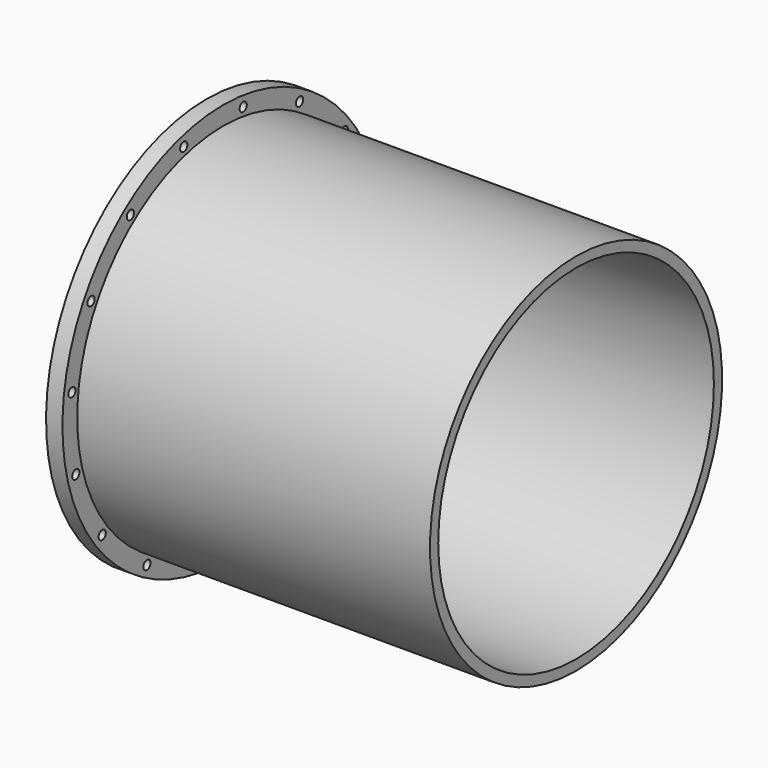
from build123d import *

# Parameters (mm, degrees)
F0_W            = 790
F0_H            = 6
F2_W            = 790
F2_H            = 8
F5_D            = 22
F5_COPIES_COUNT = 16


# Not quite as in the source:
# - a pattern or mirror of a feature is missing from the dataset's text; its kind, count and spacing are read off the source's solid


with BuildPart() as f1:
    # F0 (on Front) → F1 (revolve)
    with BuildSketch(Plane.XZ):
        Polygon((-450, 490), (-450, 420), (450, 420), (450, 445), (-410, 445), (-410, 490), align=None)
        with Locations((-15, 435)):
            Rectangle(F0_W, F0_H, mode=Mode.SUBTRACT)
    revolve(axis=Axis((-71.5964585543, 0, 0), (1, 0, 0)))

    # F2 (on Front) → F3 (revolve, cut)
    with BuildSketch(Plane.XZ):
        with Locations((-15, 434)):
            Rectangle(F2_W, F2_H)
    revolve(axis=Axis((-160.7926189899, 0, 0), (1, 0, 0)), mode=Mode.SUBTRACT)

    # F5 (through all)
    with Locations(Plane(origin=(-450, 0, 0), x_dir=(0, -1, 0), z_dir=(-1, 0, 0))):
        with Locations((-232.5, 402.7018127598)):
            f5 = Hole(F5_D / 2)

    # F5_copies: F5 ×16 about axis
    f5_copies_axis = Axis((0, 0, 0), (1, 0, 0))
    for i in range(1, F5_COPIES_COUNT):
        add(f5.rotate(f5_copies_axis, i * 360 / F5_COPIES_COUNT), mode=Mode.SUBTRACT)


solid = f1.part
